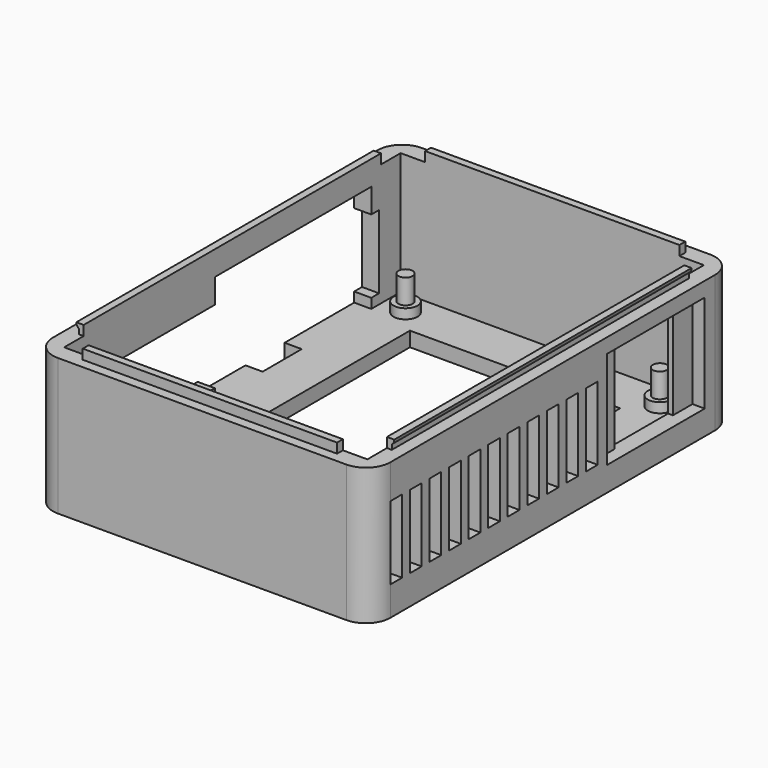
from build123d import *

# Parameters (mm, degrees)
F0_W      = 59
F0_H      = 83
F0_W_2    = 43
F0_H_2    = 67
F1_DEPTH  = 3
F2_R      = 1.45
F3_DEPTH  = 7
F4_W      = 69
F4_H      = 93
F4_W_2    = 59
F4_H_2    = 83
F5_DEPTH  = 28
F6_R      = 2.45
F7_DEPTH  = 2
F9_DEPTH  = 5
F10_W     = 15
F10_H     = 20
F10_W_2   = 3
F10_H_2   = 15
F11_DEPTH = 5
F12_W     = 62
F12_H     = 86
F12_R     = 2.5
F13_DEPTH = 25
F15_W     = 10
F15_H     = 3
F16_DEPTH = 3.5
F17_W     = 25
F17_H     = 20
F18_DEPTH = 2.5
F21_DEPTH = 76
F23_W     = 1.5
F23_H     = 2
F24_DEPTH = 52
F25_R     = 4.99999


# Not quite as in the source:
# - a fillet or chamfer is up to 0.001 mm smaller than in the source, because OpenCascade refuses the exact size


with BuildPart() as f1:
    # F0 (on Top) → F1 (new body)
    with BuildSketch(Plane.XY):
        with Locations((29.5, 41.5)):
            Rectangle(F0_W, F0_H)
        with Locations((29.5, 41.5)):
            Rectangle(F0_W_2, F0_H_2, mode=Mode.SUBTRACT)
    extrude(amount=F1_DEPTH)

    # F2 (on face) → F3 (join)
    with BuildSketch(Plane.XY.offset(3)):
        with Locations((3.5, 3.5)):
            Circle(F2_R)
        with Locations((55.5, 3.5)):
            Circle(F2_R)
        with Locations((3.5, 79.5)):
            Circle(F2_R)
        with Locations((55.5, 79.5)):
            Circle(F2_R)
    extrude(amount=F3_DEPTH)

    # F4 (on Top) → F5 (join)
    with BuildSketch(Plane.XY):
        with Locations((29.5, 41.5)):
            Rectangle(F4_W, F4_H)
        with Locations((29.5, 41.5)):
            Rectangle(F4_W_2, F4_H_2, mode=Mode.SUBTRACT)
    extrude(amount=F5_DEPTH)

    # F6 (on face) → F7 (join)
    with BuildSketch(Plane.XY.offset(3)):
        with Locations((3.5, 79.5)):
            Circle(F6_R)
        with Locations((55.5, 79.5)):
            Circle(F6_R)
        with Locations((55.5, 3.5)):
            Circle(F6_R)
        with Locations((3.5, 3.5)):
            Circle(F6_R)
    extrude(amount=F7_DEPTH)

    # F8 (on face) → F9 (cut, through all)
    with BuildSketch(Plane(origin=(-5, 0, 0), x_dir=(0, -1, 0), z_dir=(-1, 0, 0))):
        Polygon((-79, 20), (-79, 5), (-77, 5), (-77, 3), (-37, 3), (-37, 5), (-4, 5), (-4, 20), (-37, 20), (-37, 25), (-77, 25), (-77, 20), align=None)
    extrude(amount=-F9_DEPTH, mode=Mode.SUBTRACT)

    # F10 (on face) → F11 (cut, through all)
    with BuildSketch(Plane.YZ.offset(64)):
        with Locations((67.85, 15)):
            Rectangle(F10_W, F10_H)
        with Locations((1.5, 13.5)):
            Rectangle(F10_W_2, F10_H_2)
        with Locations((6.5, 13.5)):
            Rectangle(F10_W_2, F10_H_2)
        with Locations((11.5, 13.5)):
            Rectangle(F10_W_2, F10_H_2)
        with Locations((16.5, 13.5)):
            Rectangle(F10_W_2, F10_H_2)
        with Locations((21.5, 13.5)):
            Rectangle(F10_W_2, F10_H_2)
        with Locations((26.5, 13.5)):
            Rectangle(F10_W_2, F10_H_2)
        with Locations((31.5, 13.5)):
            Rectangle(F10_W_2, F10_H_2)
        with Locations((36.5, 13.5)):
            Rectangle(F10_W_2, F10_H_2)
        with Locations((41.5, 13.5)):
            Rectangle(F10_W_2, F10_H_2)
        with Locations((46.5, 13.5)):
            Rectangle(F10_W_2, F10_H_2)
        with Locations((51.5, 13.5)):
            Rectangle(F10_W_2, F10_H_2)
    extrude(amount=-F11_DEPTH, mode=Mode.SUBTRACT)

    # F12 (on face) → F13 (cut)
    with BuildSketch(Plane.XY.offset(3)):
        with Locations((29.5, 41.5)):
            Rectangle(F12_W, F12_H)
        with Locations((3.5, 3.5)):
            Circle(F12_R, mode=Mode.SUBTRACT)
        with Locations((55.5, 3.5)):
            Circle(F12_R, mode=Mode.SUBTRACT)
        with Locations((3.5, 79.5)):
            Circle(F12_R, mode=Mode.SUBTRACT)
        with Locations((55.5, 79.5)):
            Circle(F12_R, mode=Mode.SUBTRACT)
    extrude(amount=F13_DEPTH, mode=Mode.SUBTRACT)

    # F15 (on face) → F16 (cut)
    with BuildSketch(Plane(origin=(-5, 0, 0), x_dir=(0, -1, 0), z_dir=(-1, 0, 0))):
        with Locations((-54.22, 1.5)):
            Rectangle(F15_W, F15_H)
    extrude(amount=-F16_DEPTH, mode=Mode.SUBTRACT)

    # F17 (on face) → F18 (cut)
    with BuildSketch(Plane.YZ.offset(64)):
        with Locations((67.85, 15)):
            Rectangle(F17_W, F17_H)
    extrude(amount=-F18_DEPTH, mode=Mode.SUBTRACT)

    # F20 (on offset) → F21 (join)
    with BuildSketch(Plane.XZ.offset(-79.5)):
        with BuildLine():
            Line((-2.5, 29), (-2.5, 28))
            Line((-2.5, 28), (-1.5, 28))
            Line((-1.5, 28), (-1.5, 30))
            Line((-1.5, 30), (-3, 30))
            ThreePointArc((-3, 30), (-2.8716037917, 29.4391981041), (-2.5, 29))
        make_face()
        with BuildLine():
            Line((60.5, 28), (61.5, 28))
            Line((61.5, 28), (61.5, 29))
            ThreePointArc((61.5, 29), (61.8716037917, 29.4391981041), (62, 30))
            Line((62, 30), (60.5, 30))
            Line((60.5, 30), (60.5, 28))
        make_face()
    extrude(amount=F21_DEPTH)

    # F23 (on offset) → F24 (join)
    with BuildSketch(Plane.YZ.offset(3.5)):
        with Locations((-2.25, 29)):
            Rectangle(F23_W, F23_H)
        with Locations((85.25, 29)):
            Rectangle(F23_W, F23_H)
    extrude(amount=F24_DEPTH)

    # F25 (radius 5 in the source; OpenCascade refuses exactly that, so slightly less here)
    f25_edges = [f1.edges().sort_by_distance(p)[0] for p in [
        (-5, -5, 14),
        (64, -5, 14),
        (64, 88, 14),
        (-5, 88, 14),
    ]]
    fillet(f25_edges, radius=F25_R)


solid = f1.part
